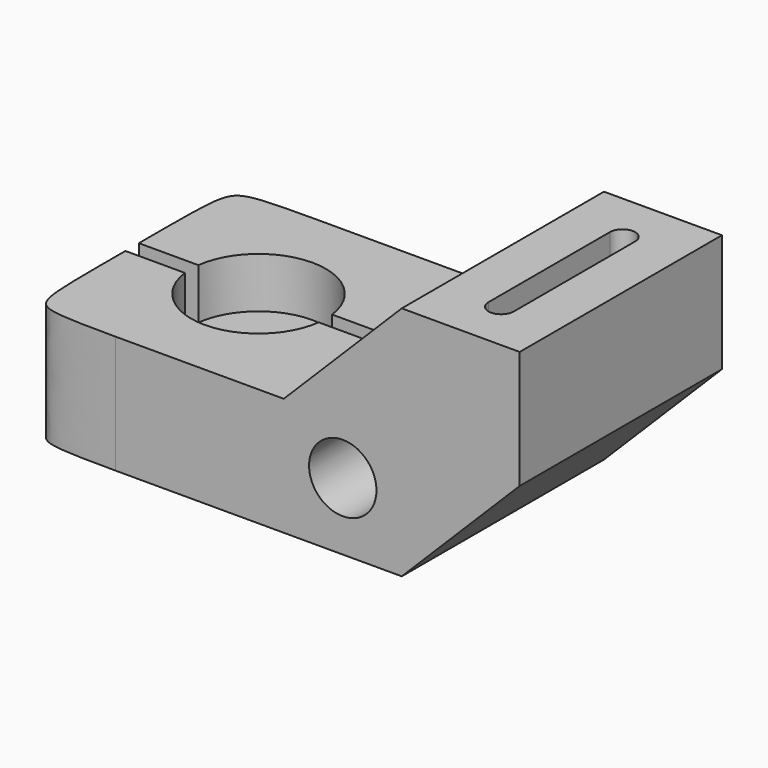
from build123d import *

# Parameters (mm, degrees)
F1_DEPTH     = 76.2
F2_R         = 10.16
F3_DEPTH     = 76.2
F5_DEPTH     = 27.94
F7_DEPTH     = 15.24
F8_R         = 7.62
F9_DEPTH     = 10.16
F10_T1_DEPTH = 162.56
F11_T1_DEPTH = 162.56


# Not quite as in the source:
# - a fillet or chamfer that OpenCascade refuses, or shapes differently, is made with other operations: its cross-section is extruded or revolved along the edge and cut away or added


with BuildPart() as f1:
    # F0 (on Front) → F1 (new body)
    with BuildSketch(Plane.XZ):
        Polygon((0, 35.56), (0, 0), (111.76, 0), (147.32, 35.56), (147.32, 71.12), (111.76, 71.12), (76.2, 35.56), align=None)
    extrude(amount=F1_DEPTH)

    # F2 (on face) → F3 (cut)
    with BuildSketch(Plane.XZ.offset(76.2)):
        with Locations((93.98, 20.32)):
            Circle(F2_R)
    extrude(amount=-F3_DEPTH, mode=Mode.SUBTRACT)

    # F4 (on face) → F5 (cut)
    with BuildSketch(Plane.XY.offset(71.12)):
        with BuildLine():
            ThreePointArc((133.35, -15.24), (129.54, -11.43), (125.73, -15.24))
            Line((125.73, -15.24), (125.73, -60.96))
            ThreePointArc((125.73, -60.96), (129.54, -64.77), (133.35, -60.96))
            Line((133.35, -60.96), (133.35, -15.24))
        make_face()
    extrude(amount=-F5_DEPTH, mode=Mode.SUBTRACT)

    # F6 (on face) → F7 (cut)
    with BuildSketch(Plane.XY.offset(35.56)):
        with BuildLine():
            ThreePointArc((58.2606249903, -40.64), (58.3801171077, -39.3724975829), (58.42, -38.1))
            ThreePointArc((58.42, -38.1), (58.3801171077, -36.8275024171), (58.2606249903, -35.56))
            ThreePointArc((58.2606249903, -35.56), (38.1, -17.78), (17.9393750097, -35.56))
            ThreePointArc((17.9393750097, -35.56), (17.78, -38.1), (17.9393750097, -40.64))
            ThreePointArc((17.9393750097, -40.64), (38.1, -58.42), (58.2606249903, -40.64))
        make_face()
        with BuildLine():
            ThreePointArc((58.2606249903, -35.56), (58.3801171077, -36.8275024171), (58.42, -38.1))
            ThreePointArc((58.42, -38.1), (58.3801171077, -39.3724975829), (58.2606249903, -40.64))
            Line((58.2606249903, -40.64), (76.2, -40.64))
            Line((76.2, -40.64), (76.2, -35.56))
            Line((76.2, -35.56), (58.2606249903, -35.56))
        make_face()
        with BuildLine():
            ThreePointArc((17.9393750097, -40.64), (17.78, -38.1), (17.9393750097, -35.56))
            Line((17.9393750097, -35.56), (0, -35.56))
            Line((0, -35.56), (0, -40.64))
            Line((0, -40.64), (17.9393750097, -40.64))
        make_face()
    extrude(amount=-F7_DEPTH, mode=Mode.SUBTRACT)

    # F8 (on face) → F9 (cut)
    with BuildSketch(Plane.XY.offset(20.32)):
        with Locations((38.1, -38.1)):
            Circle(F8_R)
    extrude(amount=-F9_DEPTH, mode=Mode.SUBTRACT)

    # F10: fillet of radius 25.4 on 1 edges, made by hand

    # F10_s2 → F10_t1 (cut)
    with BuildSketch(Plane.XY.offset(-63.5)):
        with BuildLine():
            add(Edge.make_bspline(
                [(0, -50.8), (0, -76.2), (25.4, -76.2)],
                knots=[0, 0, 0, 1, 1, 1], degree=2, weights=[1, 4, 1]))
            Line((25.4, -76.2), (0, -76.2))
            Line((0, -76.2), (0, -50.8))
        make_face()
    extrude(amount=F10_T1_DEPTH, mode=Mode.SUBTRACT)

    # F11: fillet of radius 25.4 on 1 edges, made by hand

    # F11_s2 → F11_t1 (cut)
    with BuildSketch(Plane.XY.offset(-63.5)):
        with BuildLine():
            add(Edge.make_bspline(
                [(0, -25.4), (0, 0), (25.4, 0)],
                knots=[0, 0, 0, 1, 1, 1], degree=2, weights=[1, 4, 1]))
            Line((25.4, 0), (0, 0))
            Line((0, 0), (0, -25.4))
        make_face()
    extrude(amount=F11_T1_DEPTH, mode=Mode.SUBTRACT)


solid = f1.part
